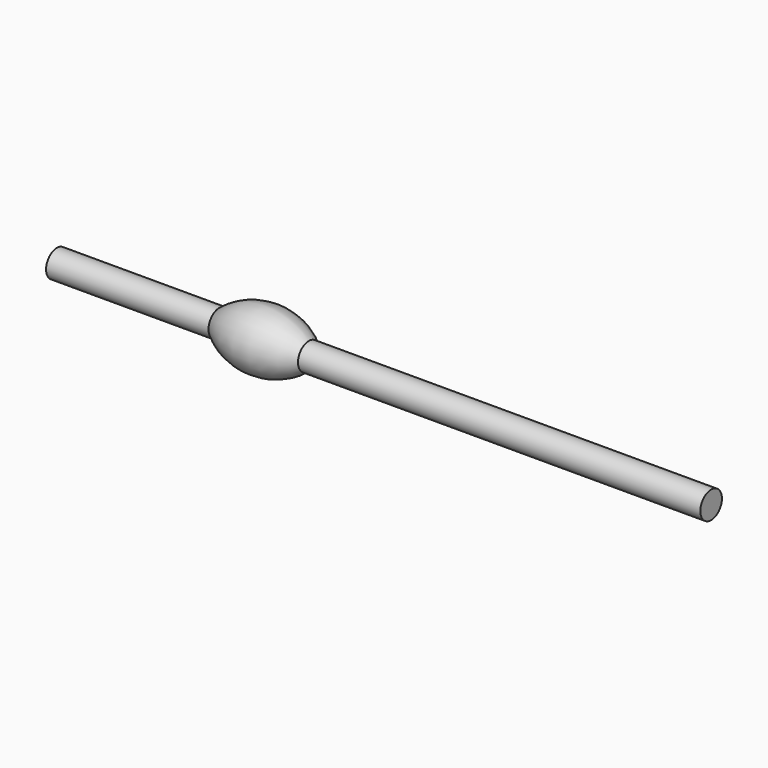
from build123d import *

# Parameters (mm, degrees)
F2_DEPTH = 305
F3_DEPTH = 75


with BuildPart() as f1:
    # F0 (on Front) → F1 (revolve)
    with BuildSketch(Plane.XZ):
        with BuildLine():
            Line((400, 0), (0, 0))
            Line((0, 0), (0, -27))
            Line((0, -27), (1079.1214704514, -27))
            Line((1079.1214704514, -27), (1079.1214704514, 0))
            Line((1079.1214704514, 0), (579.1214704514, 0))
            ThreePointArc((579.1214704514, 0), (489.5607352257, 32.3948202648), (400, 0))
        make_face()
    revolve(axis=Axis((539.5607352257, 0, -27), (1, 0, 0)))

    # F2 (add): a face of the model
    f2_faces = [f1.faces().sort_by_distance(p)[0] for p in [
        (1079.1214704514, 0, -27),
    ]]
    extrude(f2_faces, amount=F2_DEPTH)

    # F3 (cut): a face of the model
    f3_faces = [f1.faces().sort_by_distance(p)[0] for p in [
        (0, 0, -27),
    ]]
    extrude(f3_faces, amount=-F3_DEPTH, mode=Mode.SUBTRACT)


solid = f1.part
